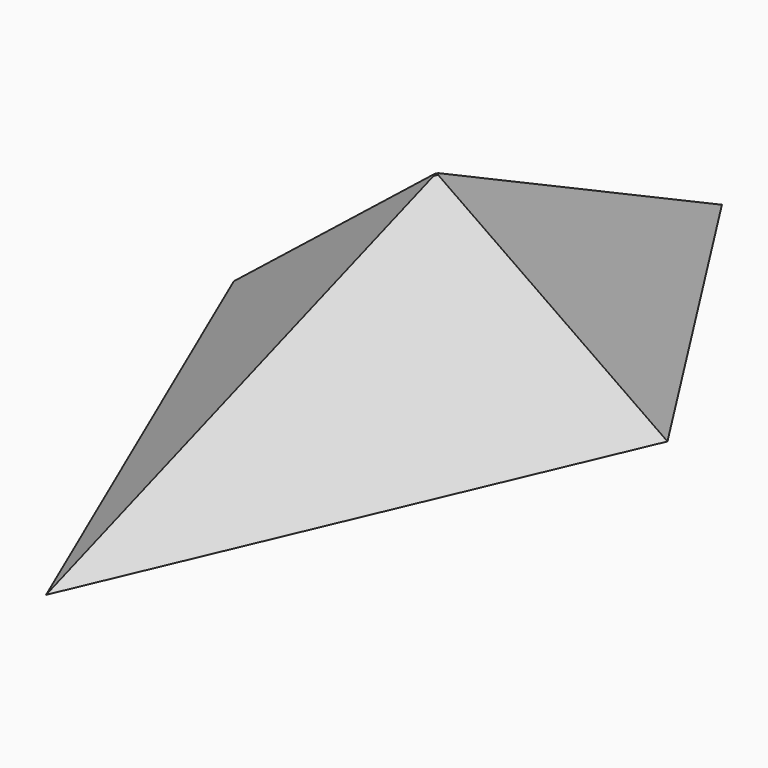
from build123d import *

# Parameters (mm, degrees)
F1_DEPTH    = 12.7
F2_T1_DEPTH = 115.269941864
F2_T3_DEPTH = 104.1696304448
F2_T5_DEPTH = 104.1696304448
F2_T7_DEPTH = 115.269941864
F3_T        = -1.905


# Not quite as in the source:
# - a fillet or chamfer that OpenCascade refuses, or shapes differently, is made with other operations: its cross-section is extruded or revolved along the edge and cut away or added


with BuildPart() as f1:
    # F0 (on Top) → F1 (new body)
    with BuildSketch(Plane.XY):
        Polygon((16.3001076085, 0), (0, 25.4906731501), (-16.3001076085, 0), (0, -38.0093268499), align=None)
    extrude(amount=F1_DEPTH)

    # F2: chamfer of 14.351 x 12.9216984397 on 4 edges, made by hand

    # F2_s2 → F2_t1 (cut)
    with BuildSketch(Plane(origin=(-28.3337655113, -66.0699536514, 0), x_dir=(0, 0, 1), z_dir=(0.3941316562, 0.9190539906, 0))):
        Polygon((-0.2216984397, 14.980678944), (12.7, 0.629678944), (12.7, 14.980678944), align=None)
    extrude(amount=F2_T1_DEPTH, mode=Mode.SUBTRACT)

    # F2_s4 → F2_t3 (cut)
    with BuildSketch(Plane(origin=(24.6401842719, -38.5331740573, 0), x_dir=(0, 0, 1), z_dir=(-0.5387272021, 0.8424802679, 0))):
        Polygon((-0.2216984397, 13.7325190245), (12.7, -0.6184809755), (12.7, 13.7325190245), align=None)
    extrude(amount=F2_T3_DEPTH, mode=Mode.SUBTRACT)

    # F2_s6 → F2_t5 (cut)
    with BuildSketch(Plane(origin=(31.4788292763, 49.227684105, 0), x_dir=(0, 0, 1), z_dir=(-0.5387272021, -0.8424802679, 0))):
        Polygon((-0.2216984397, 13.7325190245), (12.7, -0.6184809755), (12.7, 13.7325190245), align=None)
    extrude(amount=F2_T5_DEPTH, mode=Mode.SUBTRACT)

    # F2_s8 → F2_t7 (cut)
    with BuildSketch(Plane(origin=(-17.0977675905, 39.8693464092, 0), x_dir=(0, 0, 1), z_dir=(0.3941316562, -0.9190539906, 0))):
        Polygon((-0.2216984397, 14.980678944), (12.7, 0.629678944), (12.7, 14.980678944), align=None)
    extrude(amount=F2_T7_DEPTH, mode=Mode.SUBTRACT)

    # F3
    f3_openings = [f1.faces().sort_by_distance(p)[0] for p in [
        (0, -4.124591, 0),
    ]]
    offset(amount=F3_T, openings=f3_openings)


solid = f1.part
